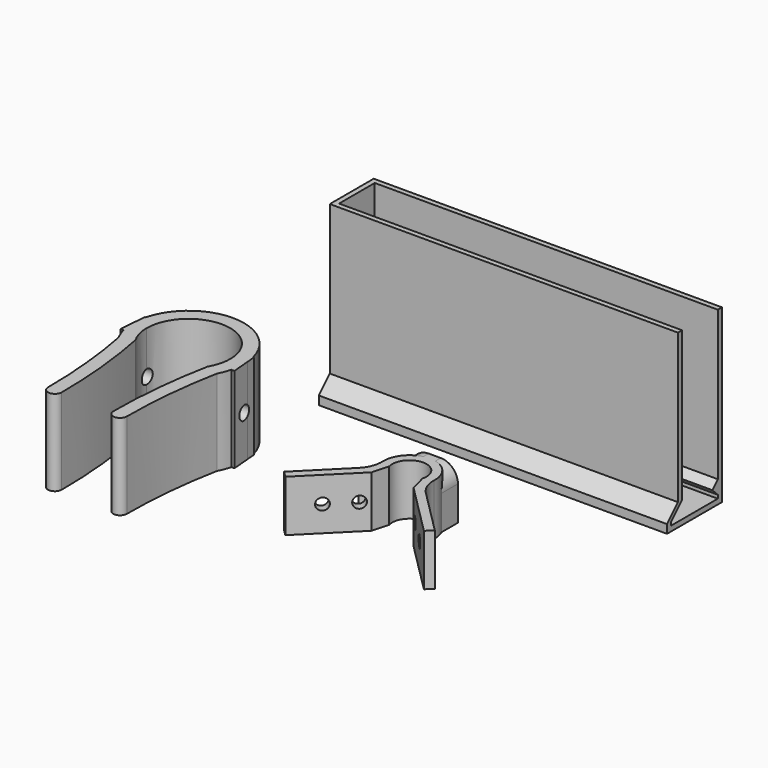
from build123d import *

# Parameters (mm, degrees)
F1_DEPTH         = 25
F2_R             = 2
F3_DEPTH         = 50
F3_DEPTH_BACK    = 25
F5_DEPTH         = 15
F6_R             = 5.25
F6_R_2           = 1.5
F7_DEPTH         = 2
F8_DEPTH         = 4.4635371399
F9_R             = 8
F10_T1_DEPTH     = 34.1738160091
F11_R            = 5
F14_D            = 3.4
F14_DEPTH        = 33.751
F14_ON_F12_D     = 3.4
F14_ON_F12_DEPTH = 32.9564066504
F16_DEPTH        = 100
F16_DEPTH_BACK   = 1.5
F17_DEPTH        = 100


# Not quite as in the source:
# - a fillet or chamfer that OpenCascade refuses, or shapes differently, is made with other operations: its cross-section is extruded or revolved along the edge and cut away or added


with BuildPart() as f1:
    # F0 (on Top) → F1 (new body)
    with BuildSketch(Plane.XY):
        with BuildLine():
            ThreePointArc((-24.161032021, 14.5729538053), (-25.4131452814, 17.5465819672), (-25.8405137163, 20.7446451753))
            ThreePointArc((-25.8405137163, 20.7446451753), (-26.8423631476, 18.0967982826), (-29.3460602999, 16.7753233416))
            ThreePointArc((-29.3460602999, 16.7753233416), (-28.7627184296, 14.9382094746), (-27.9650444616, 13.1835039897))
            ThreePointArc((-27.9650444616, 13.1835039897), (-25.8636381782, -1.3750118355), (-25.161032021, -16.0676166415))
            ThreePointArc((-25.161032021, -16.0676166415), (-23.161032021, -18.0676166415), (-21.161032021, -16.0676166415))
            ThreePointArc((-21.161032021, -16.0676166415), (-21.9128208792, -0.6740745109), (-24.161032021, 14.5729538053))
        make_face()
        with BuildLine():
            ThreePointArc((2.0239962578, 16.7753233416), (-0.4797008945, 18.0967982826), (-1.4815503258, 20.7446451753))
            ThreePointArc((-1.4815503258, 20.7446451753), (-1.9089187607, 17.5465819672), (-3.161032021, 14.5729538053))
            ThreePointArc((-3.161032021, 14.5729538053), (-5.4092431629, -0.6740745109), (-6.161032021, -16.0676166415))
            ThreePointArc((-6.161032021, -16.0676166415), (-4.161032021, -18.0676166415), (-2.161032021, -16.0676166415))
            ThreePointArc((-2.161032021, -16.0676166415), (-1.4584258639, -1.3750118355), (0.6429804195, 13.1835039897))
            ThreePointArc((0.6429804195, 13.1835039897), (1.4406543875, 14.9382094746), (2.0239962578, 16.7753233416))
        make_face()
        with BuildLine():
            ThreePointArc((-29.3460602999, 24.7139670089), (-26.8423631476, 23.392492068), (-25.8405137163, 20.7446451753))
            ThreePointArc((-25.8405137163, 20.7446451753), (-13.661032021, 32.9241268706), (-1.4815503258, 20.7446451753))
            ThreePointArc((-1.4815503258, 20.7446451753), (-0.4797008945, 23.392492068), (2.0239962578, 24.7139670089))
            ThreePointArc((2.0239962578, 24.7139670089), (-13.661032021, 36.9241268706), (-29.3460602999, 24.7139670089))
        make_face()
        with BuildLine():
            ThreePointArc((2.2312015307, 24.7343179067), (2.1274664624, 24.7254908302), (2.0239962578, 24.7139670089))
            ThreePointArc((2.0239962578, 24.7139670089), (2.2918404856, 23.4430681803), (2.4568818303, 22.1547802787))
            Line((2.4568818303, 22.1547802787), (2.2312015307, 24.7343179067))
        make_face()
        with BuildLine():
            ThreePointArc((-29.7789459209, 22.1547797242), (-29.6139045741, 23.4430679059), (-29.3460602999, 24.7139670089))
            ThreePointArc((-29.3460602999, 24.7139670089), (-29.4495305044, 24.7254908302), (-29.5532655728, 24.7343179067))
            Line((-29.5532655728, 24.7343179067), (-29.7789459209, 22.1547797242))
        make_face()
        with BuildLine():
            ThreePointArc((-30.2504289168, 16.7657044207), (-29.7979718734, 16.7448714077), (-29.3460602999, 16.7753233416))
            ThreePointArc((-29.3460602999, 16.7753233416), (-29.7883820994, 19.4468750185), (-29.7789459209, 22.1547797242))
            Line((-29.7789459209, 22.1547797242), (-30.2504289168, 16.7657044207))
        make_face()
        with BuildLine():
            ThreePointArc((2.4568818303, 22.1547802787), (2.4663180796, 19.4468752959), (2.0239962578, 16.7753233416))
            ThreePointArc((2.0239962578, 16.7753233416), (2.4759078313, 16.7448714077), (2.9283648747, 16.7657044207))
            Line((2.9283648747, 16.7657044207), (2.4568818303, 22.1547802787))
        make_face()
        with BuildLine():
            ThreePointArc((2.0239962578, 24.7139670089), (-0.4797008945, 23.392492068), (-1.4815503258, 20.7446451753))
            ThreePointArc((-1.4815503258, 20.7446451753), (-0.4797008945, 18.0967982826), (2.0239962578, 16.7753233416))
            ThreePointArc((2.0239962578, 16.7753233416), (2.4663180796, 19.4468752959), (2.4568818303, 22.1547802787))
            ThreePointArc((2.4568818303, 22.1547802787), (2.2918404856, 23.4430681803), (2.0239962578, 24.7139670089))
        make_face()
        with BuildLine():
            ThreePointArc((-29.3460602999, 16.7753233416), (-26.8423631476, 18.0967982826), (-25.8405137163, 20.7446451753))
            ThreePointArc((-25.8405137163, 20.7446451753), (-26.8423631476, 23.392492068), (-29.3460602999, 24.7139670089))
            ThreePointArc((-29.3460602999, 24.7139670089), (-29.6139045741, 23.4430679059), (-29.7789459209, 22.1547797242))
            ThreePointArc((-29.7789459209, 22.1547797242), (-29.7883820994, 19.4468750185), (-29.3460602999, 16.7753233416))
        make_face()
    extrude(amount=F1_DEPTH)

    # F2 (on Right) → F3 (cut, two sides)
    with BuildSketch(Plane.YZ) as f3_sk:
        with Locations((20.7500111637, 12.5)):
            Circle(F2_R)
    extrude(amount=-F3_DEPTH, mode=Mode.SUBTRACT)
    extrude(f3_sk.sketch, amount=F3_DEPTH_BACK, mode=Mode.SUBTRACT)


with BuildPart() as f5:
    # F4 (on Top) → F5 (new body)
    with BuildSketch(Plane.XY):
        with BuildLine():
            Line((30.8044720441, 0), (32.5722389971, -1.767766953))
            Line((32.5722389971, -1.767766953), (49.1261838352, 14.7861778852))
            ThreePointArc((49.1261838352, 14.7861778852), (52.6617177411, 23.3217117911), (56.1972516471, 14.7861778852))
            Line((56.1972516471, 14.7861778852), (73.8749211767, -2.8914916445))
            Line((73.8749211767, -2.8914916445), (75.6426881297, -1.1237246915))
            Line((75.6426881297, -1.1237246915), (59.4294846941, 15.0894787441))
            ThreePointArc((59.4294846941, 15.0894787441), (60.1617177411, 18.3217117911), (59.4294846941, 21.5539448381))
            ThreePointArc((59.4294846941, 21.5539448381), (56.6622334671, 24.6656753728), (52.6617177411, 25.8217117911))
            ThreePointArc((52.6617177411, 25.8217117911), (48.6612020152, 24.6656753728), (45.8939507882, 21.5539448381))
            ThreePointArc((45.8939507882, 21.5539448381), (45.1617177411, 18.3217117911), (45.8939507882, 15.0894787441))
            Line((45.8939507882, 15.0894787441), (30.8044720441, 0))
        make_face()
        with BuildLine():
            Line((45.8939507882, 25.8217117911), (45.8939507882, 21.5539448381))
            ThreePointArc((45.8939507882, 21.5539448381), (48.6612020152, 24.6656753728), (52.6617177411, 25.8217117911))
            Line((52.6617177411, 25.8217117911), (45.8939507882, 25.8217117911))
        make_face()
        with BuildLine():
            Line((45.8939507882, 25.8217117911), (52.6617177411, 25.8217117911))
            ThreePointArc((52.6617177411, 25.8217117911), (56.6622334671, 24.6656753728), (59.4294846941, 21.5539448381))
            Line((59.4294846941, 21.5539448381), (59.4294846941, 27.5539448381))
            Line((59.4294846941, 27.5539448381), (45.8939507882, 27.5539448381))
            Line((45.8939507882, 27.5539448381), (45.8939507882, 25.8217117911))
        make_face()
    extrude(amount=F5_DEPTH)

    # F6 (on face) → F7 (cut)
    with BuildSketch(Plane(origin=(0, 27.5539448381, 0), x_dir=(-1, 0, 0), z_dir=(0, 1, 0))):
        with Locations((-52.6617177411, 7.5)):
            Circle(F6_R)
        with Locations((-52.6617177411, 7.5)):
            Circle(F6_R_2, mode=Mode.SUBTRACT)
    extrude(amount=-F7_DEPTH, mode=Mode.SUBTRACT)

    # F8 (cut, through all): a face of the model
    f8_faces = [f5.faces().sort_by_distance(p)[0] for p in [
        (52.6617177411, 27.5539448381, 7.5),
    ]]
    extrude(f8_faces, amount=-F8_DEPTH, mode=Mode.SUBTRACT)

    # F9
    f9_edges = [f5.edges().sort_by_distance(p)[0] for p in [
        (59.429485, 15.089479, 7.5),
        (45.893951, 15.089479, 7.5),
    ]]
    fillet(f9_edges, radius=F9_R)

    # F10: chamfer of 5 on 2 edges, made by hand

    # F10_s2 → F10_t1 (cut)
    with BuildSketch(Plane.XY.offset(-9.5869080045)):
        with BuildLine():
            Line((58.7854420981, 12.1979874341), (57.4913468726, 17.0276165656))
            ThreePointArc((57.4913468726, 17.0276165656), (57.0285091449, 15.8863200699), (56.1972516471, 14.7861778852))
            Line((56.1972516471, 14.7861778852), (58.7854420981, 12.1979874341))
        make_face()
        with BuildLine():
            Line((47.8320886097, 17.0276165656), (46.5379933842, 12.1979874341))
            Line((46.5379933842, 12.1979874341), (49.1261838352, 14.7861778852))
            ThreePointArc((49.1261838352, 14.7861778852), (48.2949263373, 15.8863200699), (47.8320886097, 17.0276165656))
        make_face()
    extrude(amount=F10_T1_DEPTH, mode=Mode.SUBTRACT)

    # F11
    f11_edges = [f5.edges().sort_by_distance(p)[0] for p in [
        (45.893951, 24.553945, 15),
        (59.429485, 24.553945, 15),
    ]]
    fillet(f11_edges, radius=F11_R)

    # F14 (through all, one way)
    with BuildSketch(Plane(origin=(15.4022360221, -15.4022360221, 0), x_dir=(-0.7071067812, -0.7071067812, 0), z_dir=(-0.7071067812, 0.7071067812, 0))):
        with Locations((-38.7911101231, 7.5), (-30.2865805982, 7.5)):
            Circle(F14_D / 2)
    extrude(amount=-F14_DEPTH, mode=Mode.SUBTRACT)

    # F14 on F12 (through all, one way)
    with BuildSketch(Plane(origin=(37.2594817191, 37.2594817191, 0), x_dir=(-0.7071067812, 0.7071067812, 0), z_dir=(0.7071067812, 0.7071067812, 0))):
        with Locations((-35.6838053243, 7.5), (-44.9829281988, 7.5)):
            Circle(F14_ON_F12_D / 2)
    extrude(amount=-F14_ON_F12_DEPTH, mode=Mode.SUBTRACT)


with BuildPart() as f16:
    # F15 (on Right) → F16 (new body, two sides)
    with BuildSketch(Plane.YZ) as f16_sk:
        Polygon((53.036596626, 2.5), (53.036596626, 0), (73.036596626, 0), (73.036596626, 50), (71.536596626, 50), (71.536596626, 6.5), (71.536596626, 4.5), (71.536596626, 2.5), (71.536596626, 1.5), (54.536596626, 1.5), (54.536596626, 2.5), (56.536596626, 4.5), (58.536596626, 6.5), (58.536596626, 50), (57.036596626, 50), (57.036596626, 6.5), align=None)
        Polygon((71.536596626, 4.5), (71.536596626, 6.5), (69.536596626, 4.5), align=None)
        Polygon((71.536596626, 2.5), (71.536596626, 4.5), (69.536596626, 4.5), align=None)
        Polygon((71.536596626, 6.5), (71.536596626, 50), (58.536596626, 50), (58.536596626, 6.5), (56.536596626, 4.5), (54.536596626, 2.5), (54.536596626, 1.5), (71.536596626, 1.5), (71.536596626, 2.5), (69.536596626, 4.5), align=None)
    extrude(amount=F16_DEPTH)
    extrude(f16_sk.sketch, amount=-F16_DEPTH_BACK)

    # F15 (on Right) → F17 (cut)
    with BuildSketch(Plane.YZ):
        Polygon((71.536596626, 6.5), (71.536596626, 50), (58.536596626, 50), (58.536596626, 6.5), (56.536596626, 4.5), (54.536596626, 2.5), (54.536596626, 1.5), (71.536596626, 1.5), (71.536596626, 2.5), (69.536596626, 4.5), align=None)
    extrude(amount=F17_DEPTH, mode=Mode.SUBTRACT)


solid = Compound([f1.part, f5.part, f16.part])
